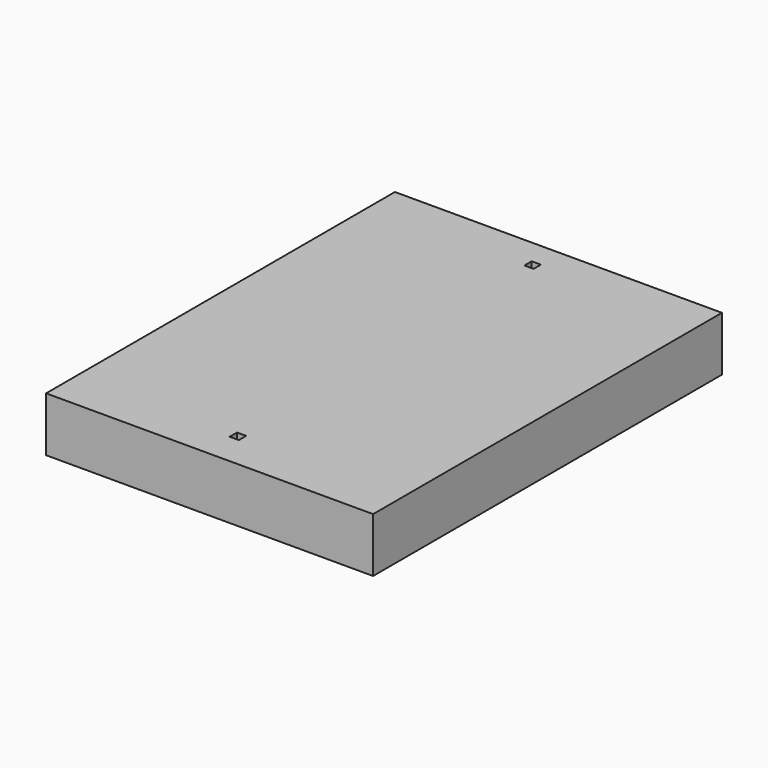
from build123d import *

# Parameters (mm, degrees)
F0_W     = 152.4
F0_H     = 203.2
F2_DEPTH = 25.4
F3_W     = 4.2672
F3_H     = 4.2672
F4_DEPTH = 25.401
F5_W     = 4.2672
F5_H     = 4.2672
F6_DEPTH = 25.401


# Not quite as in the source:
# - a feature names something its author has since deleted; it is built from what else it names


with BuildPart() as f2:
    # F0 (on Top) → F2 (new body)
    with BuildSketch(Plane.XY):
        with Locations((-31.6100876886, -2.4557895958)):
            Rectangle(F0_W, F0_H)
    extrude(amount=F2_DEPTH)

    # F3 (on face) → F4 (cut, through all)
    with BuildSketch(Plane.XY.offset(25.4)):
        with Locations((-32.6907886192, 85.4696582746)):
            Rectangle(F3_W, F3_H)
    extrude(amount=-F4_DEPTH, mode=Mode.SUBTRACT)

    # F5 (on face) → F6 (cut, through all)
    with BuildSketch(Plane.XY.offset(25.4)):
        with Locations((-32.1158650086, -86.9036130607)):
            Rectangle(F5_W, F5_H)
    extrude(amount=-F6_DEPTH, mode=Mode.SUBTRACT)


solid = f2.part
